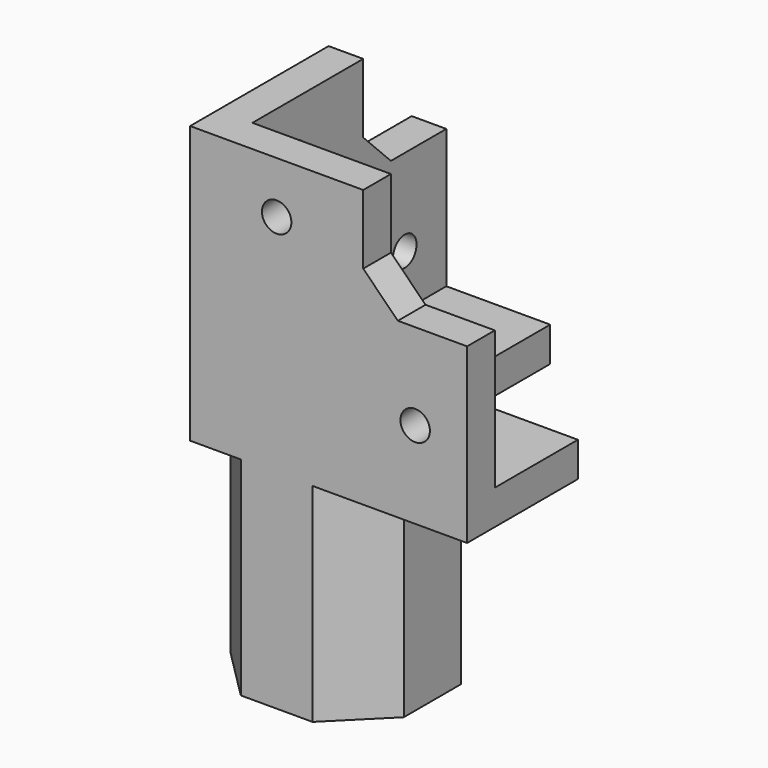
from build123d import *

# Parameters (mm, degrees)
F0_R        = 4.875
F0_R_2      = 2.125
F1_DEPTH    = 5
F2_R        = 4.875
F3_DEPTH    = 30
F4_T1_DEPTH = 5
F6_DEPTH    = 20
F8_DEPTH    = 15
F9_R        = 2.125
F10_DEPTH   = 40.001
F11_R       = 2.125
F12_DEPTH   = 40.001
F13_SIZE    = 5


# Not quite as in the source:
# - a fillet or chamfer that OpenCascade refuses, or shapes differently, is made with other operations: its cross-section is extruded or revolved along the edge and cut away or added


with BuildPart() as f1:
    # F0 (on Top) → F1 (new body)
    with BuildSketch(Plane.XY):
        Polygon((-12.5, 27.5), (-12.5, 0), (-12.5, -12.5), (27.5, -12.5), (27.5, 7.5), (7.5, 7.5), (7.5, 27.5), align=None)
        Circle(F0_R, mode=Mode.SUBTRACT)
        with Locations((17.5, 0)):
            Circle(F0_R_2, mode=Mode.SUBTRACT)
        with Locations((0, 17.5)):
            Circle(F0_R_2, mode=Mode.SUBTRACT)
    extrude(amount=F1_DEPTH)

    # F2 (on face) → F3 (join)
    with BuildSketch(Plane(origin=(0, 0, 0), x_dir=(1, 0, 0), z_dir=(0, 0, -1))):
        Polygon((12.5, -5.1776695297), (12.5, 5.1776695297), (5.1776695297, 12.5), (-5.1776695297, 12.5), (-12.5, 5.1776695297), (-12.5, -5.1776695297), (-5.1776695297, -12.5), (5.1776695297, -12.5), (7.5, -10.1776695297), (7.5, -7.5), (10.1776695297, -7.5), align=None)
        Circle(F2_R, mode=Mode.SUBTRACT)
        Polygon((7.5, -10.1776695297), (10.1776695297, -7.5), (7.5, -7.5), align=None)
    extrude(amount=F3_DEPTH)

    # F4: chamfer of 5 on 1 edges, made by hand

    # F4_s2 → F4_t1 (join)
    with BuildSketch(Plane.XY):
        Polygon((12.5, 7.5), (7.5, 12.5), (7.5, 7.5), align=None)
    extrude(amount=F4_T1_DEPTH)

    # F5 (on face) → F6 (join)
    with BuildSketch(Plane.XY.offset(5)):
        Polygon((-7.5, 27.5), (-12.5, 27.5), (-12.5, -12.5), (27.5, -12.5), (27.5, -7.5), (-7.5, -7.5), align=None)
    extrude(amount=F6_DEPTH)

    # F7 (on face) → F8 (join)
    with BuildSketch(Plane.XY.offset(25)):
        Polygon((-7.5, 12.5), (-12.5, 12.5), (-12.5, -12.5), (12.5, -12.5), (12.5, -7.5), (-7.5, -7.5), align=None)
    extrude(amount=F8_DEPTH)

    # F9 (on face) → F10 (cut, through all)
    with BuildSketch(Plane.XZ.offset(12.5)):
        with Locations((20, 12.5)):
            Circle(F9_R)
        with Locations((0, 32.5)):
            Circle(F9_R)
    extrude(amount=-F10_DEPTH, mode=Mode.SUBTRACT)

    # F11 (on face) → F12 (cut, through all)
    with BuildSketch(Plane(origin=(-12.5, 0, 0), x_dir=(0, -1, 0), z_dir=(-1, 0, 0))):
        with Locations((-20, 12.5)):
            Circle(F11_R)
        with Locations((0, 32.5)):
            Circle(F11_R)
    extrude(amount=-F12_DEPTH, mode=Mode.SUBTRACT)

    # F13
    f13_edges = [f1.edges().sort_by_distance(p)[0] for p in [
        (12.5, -10, 25),
        (-10, 12.5, 25),
    ]]
    chamfer(f13_edges, length=F13_SIZE)


solid = f1.part
